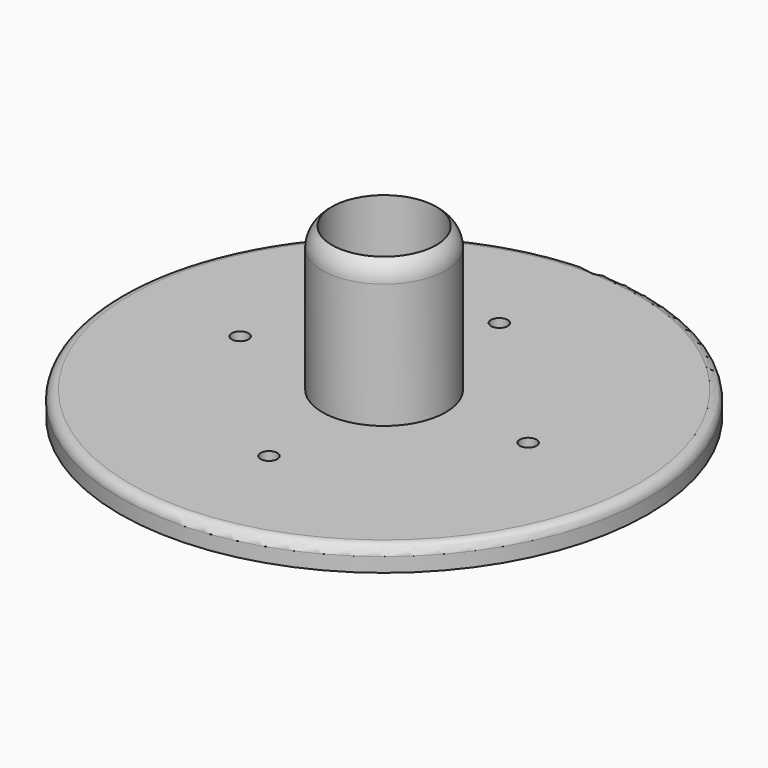
from build123d import *

# Parameters (mm, degrees)
F0_R     = 55
F1_DEPTH = 5
F2_R     = 10.85
F3_DEPTH = 25
F4_R     = 12.85
F4_R_2   = 10.85
F5_DEPTH = 30
F7_R     = 2
F8_R     = 1.75
F9_DEPTH = 25


# Not quite as in the source:
# - a fillet or chamfer that OpenCascade refuses, or shapes differently, is made with other operations: its cross-section is extruded or revolved along the edge and cut away or added


with BuildPart() as f1:
    # F0 (on Top) → F1 (new body)
    with BuildSketch(Plane.XY):
        Circle(F0_R)
    extrude(amount=F1_DEPTH)

    # F2 (on face) → F3 (cut)
    with BuildSketch(Plane.XY.offset(5)):
        Circle(F2_R)
    extrude(amount=-F3_DEPTH, mode=Mode.SUBTRACT)

    # F4 (on face) → F5 (join)
    with BuildSketch(Plane.XY.offset(5)):
        Circle(F4_R)
        Circle(F4_R_2, mode=Mode.SUBTRACT)
    extrude(amount=F5_DEPTH)

    # F6: fillet of radius 5 on 1 edges, made by hand

    # F6_s1 → F6_t2 (revolve, cut)
    with BuildSketch(Plane.XZ):
        with BuildLine():
            ThreePointArc((12.85, 31), (12.322135955, 33.2360679775), (10.85, 35))
            Line((10.85, 35), (12.85, 35))
            Line((12.85, 35), (12.85, 31))
        make_face()
    revolve(axis=Axis((0, 0, 35), (0, 0, 1)), mode=Mode.SUBTRACT)

    # F7
    f7_edges = [f1.edges().sort_by_distance(p)[0] for p in [
        (-55, 0, 5),
    ]]
    fillet(f7_edges, radius=F7_R)

    # F8 (on face) → F9 (cut)
    with BuildSketch(Plane.XY.offset(5)):
        with Locations((-30, 0)):
            Circle(F8_R)
        with Locations((0, -30)):
            Circle(F8_R)
        with Locations((30, 0)):
            Circle(F8_R)
        with Locations((0, 30)):
            Circle(F8_R)
    extrude(amount=-F9_DEPTH, mode=Mode.SUBTRACT)


solid = f1.part
